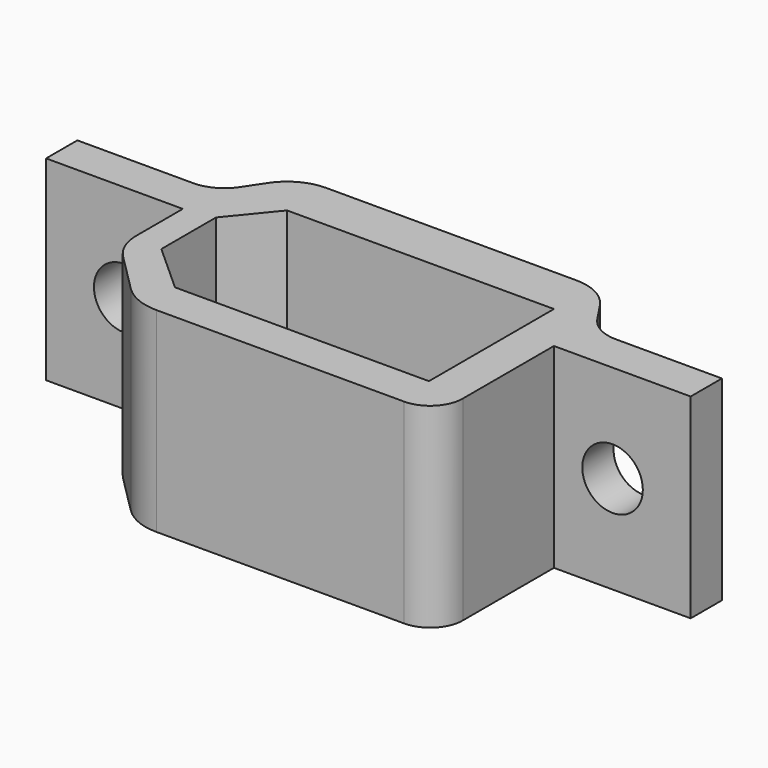
from build123d import *

# Parameters (mm, degrees)
F1_DEPTH = 10
F2_R     = 1.55
F3_DEPTH = 5
F4_R     = 3.075
F5_DEPTH = 5
F6_R     = 3.075
F7_DEPTH = 5


# Not quite as in the source:
# - a feature names something its author has since deleted; it is built from what else it names


with BuildPart() as f1:
    # F0 (on Top) → F1 (new body)
    with BuildSketch(Plane.XY):
        with BuildLine():
            Line((-1.5664058328, 14.3066409416), (-5.9960383158, 14.3066409416))
            ThreePointArc((-5.9960383158, 14.3066409416), (-6.9397541669, 14.5432917441), (-7.6601389045, 15.1972405492))
            Line((-7.6601389045, 15.1972405492), (-8.3242394931, 16.1933914322))
            ThreePointArc((-8.3242394931, 16.1933914322), (-8.8670406285, 16.7780954993), (-9.5664058328, 17.1620228746))
            ThreePointArc((-9.5664058328, 17.1620228746), (-9.9791916365, 17.2702211446), (-10.404365229, 17.3066409416))
            Line((-10.404365229, 17.3066409416), (-23.2284464365, 17.3066409416))
            ThreePointArc((-23.2284464365, 17.3066409416), (-24.4080912504, 17.0108274386), (-25.3085721724, 16.1933914322))
            Line((-25.3085721724, 16.1933914322), (-25.9726727611, 15.1972405492))
            ThreePointArc((-25.9726727611, 15.1972405492), (-26.6930574987, 14.5432917441), (-27.6367733497, 14.3066409416))
            Line((-27.6367733497, 14.3066409416), (-32.5664058328, 14.3066409416))
            Line((-32.5664058328, 14.3066409416), (-33.5664058328, 14.3066409416))
            Line((-33.5664058328, 14.3066409416), (-33.5664058328, 12.3066409416))
            Line((-33.5664058328, 12.3066409416), (-32.5664058328, 12.3066409416))
            Line((-32.5664058328, 12.3066409416), (-26.5664058328, 12.3066409416))
            Line((-26.5664058328, 12.3066409416), (-26.5664058328, 9.3240286596))
            ThreePointArc((-26.5664058328, 9.3240286596), (-26.3794394083, 8.3840849704), (-25.8470040783, 7.5872391872))
            Line((-25.8470040783, 7.5872391872), (-23.8748829035, 5.6151180124))
            ThreePointArc((-23.8748829035, 5.6151180124), (-22.979372793, 5.0167572865), (-21.9230465945, 4.8066409416))
            Line((-21.9230465945, 4.8066409416), (-9.2356068064, 4.8066409416))
            ThreePointArc((-9.2356068064, 4.8066409416), (-8.0553034788, 5.2955385877), (-7.5664058328, 6.4758419153))
            Line((-7.5664058328, 6.4758419153), (-7.5664058328, 12.3066409416))
            Line((-7.5664058328, 12.3066409416), (-1.5664058328, 12.3066409416))
            Line((-1.5664058328, 12.3066409416), (-0.5664058328, 12.3066409416))
            Line((-0.5664058328, 12.3066409416), (-0.5664058328, 14.3066409416))
            Line((-0.5664058328, 14.3066409416), (-1.5664058328, 14.3066409416))
        make_face()
        Polygon((-9.5664058328, 14.8066409416), (-9.5664058328, 6.8066409416), (-22.5664058328, 6.8066409416), (-25.0664058328, 9.0566409416), (-25.0664058328, 10.8066409416), (-25.0664058328, 12.5566409416), (-23.2284464365, 14.8066409416), (-22.5664058328, 14.8066409416), align=None, mode=Mode.SUBTRACT)
    extrude(amount=F1_DEPTH)

    # F2 (on face) → F3 (cut)
    with BuildSketch(Plane.XZ.offset(-12.3066409416)):
        with Locations((-29.5664058328, 5)):
            Circle(F2_R)
        with Locations((-4.5664058328, 5)):
            Circle(F2_R)
    extrude(amount=-F3_DEPTH, mode=Mode.SUBTRACT)

    # F4 (on face) → F5 (cut)
    with BuildSketch(Plane(origin=(0, 14.3066409416, 0), x_dir=(-1, 0, 0), z_dir=(0, 1, 0))):
        with Locations((29.5664058328, 5)):
            Circle(F4_R)
    extrude(amount=F5_DEPTH, mode=Mode.SUBTRACT)

    # F6 (on face) → F7 (cut)
    with BuildSketch(Plane(origin=(0, 14.3066409416, 0), x_dir=(-1, 0, 0), z_dir=(0, 1, 0))):
        with Locations((4.5664058328, 5)):
            Circle(F6_R)
    extrude(amount=F7_DEPTH, mode=Mode.SUBTRACT)


solid = f1.part
